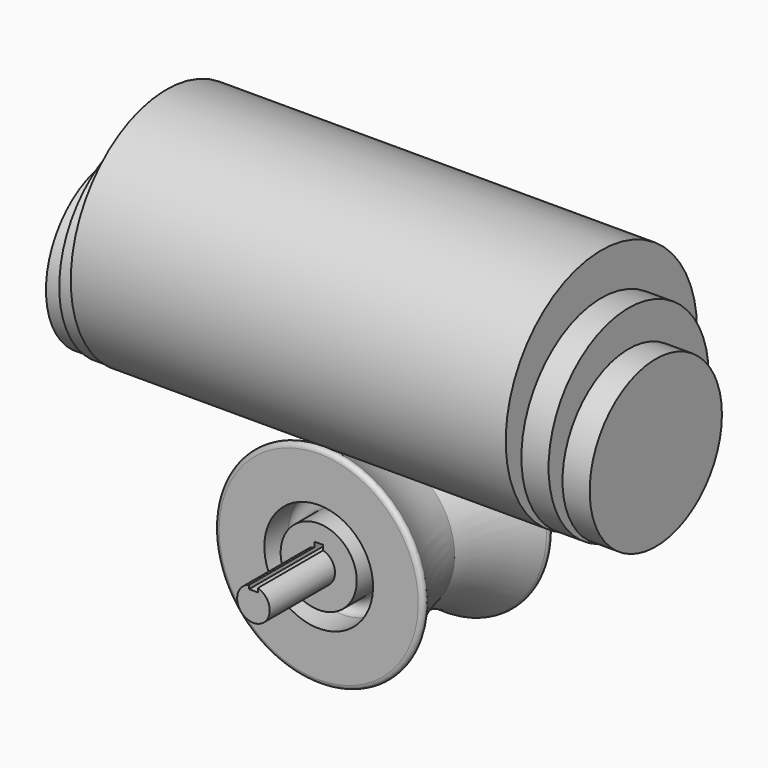
from build123d import *

# Parameters (mm, degrees)
F3_DEPTH  = 150.001
F7_DEPTH  = 112.501
F8_R      = 2
F9_R      = 38
F10_DEPTH = 125
F13_R     = 46
F14_DEPTH = 112.5
F16_R     = 55
F17_DEPTH = 100


# Not quite as in the source:
# - a feature names something its author has since deleted; it is built from what else it names


with BuildPart() as f1:
    # F0 (on Right) → F1 (revolve)
    with BuildSketch(Plane.YZ):
        Polygon((75, 7.5), (0, 7.5), (-75, 7.5), (-75, 0), (75, 0), align=None)
    revolve(axis=Axis((0, 0, 0), (0, 1, 0)))

    # F2 (on face) → F3 (cut, through all)
    with BuildSketch(Plane.XZ.offset(75)):
        with BuildLine():
            Line((2, 5.5), (2, 7.2284161474))
            ThreePointArc((2, 7.2284161474), (0, 7.5), (-2, 7.2284161474))
            Line((-2, 7.2284161474), (-2, 5.5))
            Line((-2, 5.5), (0, 5.5))
            Line((0, 5.5), (2, 5.5))
        make_face()
    extrude(amount=-F3_DEPTH, mode=Mode.SUBTRACT)


with BuildPart() as f5:
    # F4 (on Right) → F5 (revolve)
    with BuildSketch(Plane.YZ):
        with BuildLine():
            Line((-37.5, 7.5), (0, 7.5))
            Line((0, 7.5), (37.5, 7.5))
            Line((37.5, 7.5), (37.5, 17.5))
            Line((37.5, 17.5), (23.8281880061, 17.5))
            ThreePointArc((23.8281880061, 17.5), (20.0781880061, 21.25), (23.8281880061, 25))
            Line((23.8281880061, 25), (37.5, 25))
            Line((37.5, 25), (37.5, 50))
            ThreePointArc((37.5, 50), (19.9640337403, 38.648499128), (0, 32.5))
            ThreePointArc((0, 32.5), (-19.9640337403, 38.648499128), (-37.5, 50))
            Line((-37.5, 50), (-37.5, 25))
            Line((-37.5, 25), (-23.8281880061, 25))
            ThreePointArc((-23.8281880061, 25), (-20.0781880061, 21.25), (-23.8281880061, 17.5))
            Line((-23.8281880061, 17.5), (-37.5, 17.5))
            Line((-37.5, 17.5), (-37.5, 7.5))
        make_face()
    revolve(axis=Axis((0, 75, 0), (0, -1, 0)))

    # F6 (on face) → F7 (cut, through all)
    with BuildSketch(Plane.XZ.offset(37.5)):
        with BuildLine():
            Line((-2, 9.5), (-2, 7.2284161474))
            ThreePointArc((-2, 7.2284161474), (0, 7.5), (2, 7.2284161474))
            Line((2, 7.2284161474), (2, 9.5))
            Line((2, 9.5), (-2, 9.5))
        make_face()
    extrude(amount=-F7_DEPTH, mode=Mode.SUBTRACT)

    # F8
    f8_edges = [f5.edges().sort_by_distance(p)[0] for p in [
        (0, -37.5, -50),
        (0, 37.5, -50),
    ]]
    fillet(f8_edges, radius=F8_R)


with BuildPart() as f10:
    # F9 (on Right) → F10 (new body, symmetric)
    with BuildSketch(Plane.YZ):
        with Locations((0, 71.5217095242)):
            Circle(F9_R)
    extrude(amount=F10_DEPTH, both=True)


with BuildPart() as f11_1:
    # F11: copy of F10
    add(f10.part)


with BuildPart() as f14:
    # F13 (on Right) → F14 (new body, symmetric)
    with BuildSketch(Plane.YZ):
        with Locations((0, 419.790243499)):
            Circle(F13_R)
    extrude(amount=F14_DEPTH, both=True)


with BuildPart() as f14b:
    # F13 (on Right) → F14, piece 2 (new body, symmetric)
    with BuildSketch(Plane.YZ):
        with Locations((0, 80.1001208774)):
            Circle(F13_R)
    extrude(amount=F14_DEPTH, both=True)


with BuildPart() as f17:
    # F16 (on Right) → F17 (new body, symmetric)
    with BuildSketch(Plane.YZ):
        with Locations((0, 90.4080991159)):
            Circle(F16_R)
    extrude(amount=F17_DEPTH, both=True)


solid = Compound([f1.part, f5.part, f10.part, f14b.part, f17.part])
